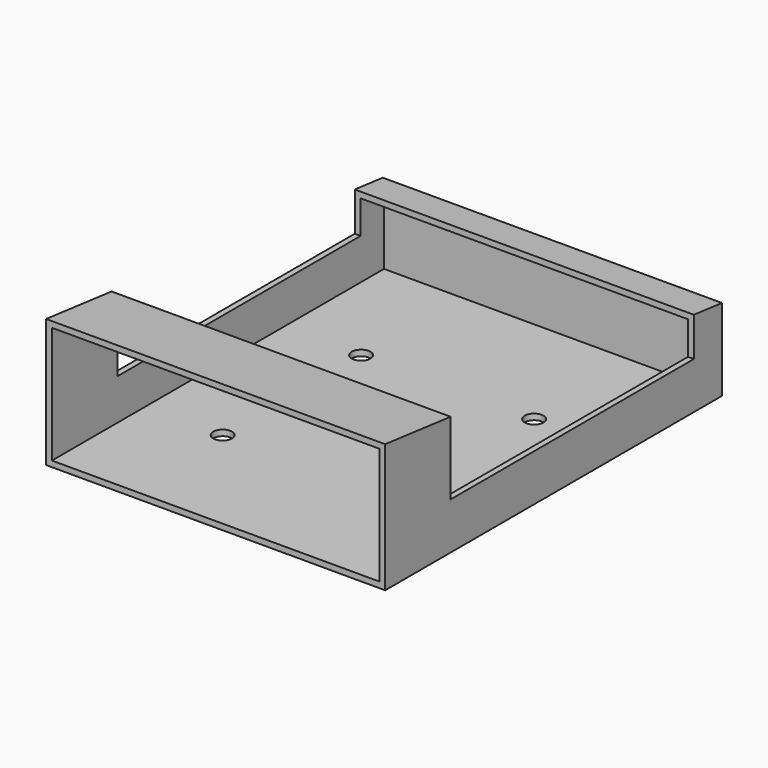
from build123d import *

# Parameters (mm, degrees)
F1_DEPTH = 145
F2_T     = -2.5
F4_DEPTH = 145
F6_D     = 8


# Not quite as in the source:
# - a feature names something its author has since deleted; it is built from what else it names


with BuildPart() as f1:
    # F0 (on Right) → F1 (new body)
    with BuildSketch(Plane.YZ):
        Polygon((109.173472161, 35), (-70.826527839, 55), (-70.826527839, 0), (109.173472161, 0), align=None)
    extrude(amount=F1_DEPTH)

    # F2
    f2_openings = [f1.faces().sort_by_distance(p)[0] for p in [
        (72.5, -70.826528, 27.5),
    ]]
    offset(amount=F2_T, openings=f2_openings)

    # F3 (on face) → F4 (cut)
    with BuildSketch(Plane.YZ.offset(145)):
        Polygon((94.173472161, 36.6666666667), (-35.826527839, 51.1111111111), (-35.826527839, 20), (94.173472161, 20), align=None)
    extrude(amount=-F4_DEPTH, mode=Mode.SUBTRACT)

    # F6 (through all)
    with Locations(Plane(origin=(0, 0, 0), x_dir=(1, 0, 0), z_dir=(0, 0, -1))):
        with Locations((109.5, 20.826527839), (35.5, 20.826527839), (35.5, -53.173472161), (109.5, -53.173472161)):
            Hole(F6_D / 2)


solid = f1.part
